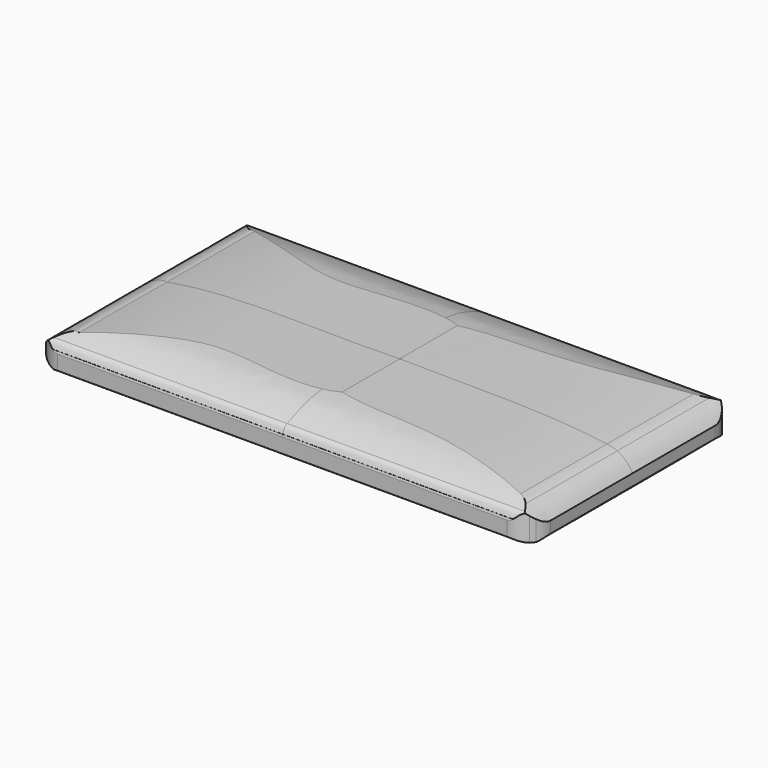
from build123d import *

# Parameters (mm, degrees)
F1_DEPTH = 40
F2_R     = 42.893475334
F3_DEPTH = 77.3
F5_DEPTH = 15


# Not quite as in the source:
# - a feature names something its author has since deleted; it is built from what else it names


with BuildPart() as f1:
    # F0 (on Front) → F1 (new body, symmetric)
    with BuildSketch(Plane.XZ):
        with BuildLine():
            add(Edge.make_bspline(
                [(72.5, -2.7491913643), (72.416496151, -3.810280827), (71.2043847412, -5.7919796052), (69.2787097317, -6.0699322478), (68.1885108352, -6.1267605634)],
                knots=[0, 0, 0, 0, 0.503951183, 1, 1, 1, 1], degree=3))
            add(Edge.make_bspline(
                [(72.5, -2.7491913643), (71.7240370512, -0.9958820883), (70.00554353, 1.4875582419), (67.2821030021, 2.8555840254)],
                knots=[0, 0, 0, 0, 7.657673031, 7.657673031, 7.657673031, 7.657673031], degree=3))
            add(Edge.make_bspline(
                [(67.2821030021, 2.8555840254), (66.6986107826, 3.1973873265), (65.1900321245, 3.5558441274), (64.3139258027, 3.6549806215)],
                knots=[0, 0, 0, 0, 3.0739405988, 3.0739405988, 3.0739405988, 3.0739405988], degree=3))
            add(Edge.make_bspline(
                [(64.3139258027, 3.6549806215), (46.5292930603, 6.1267605634), (25.1828059554, 5.4464280226), (4.5694559813, 5.8230283291)],
                knots=[0, 0, 0, 0, 59.7837946697, 59.7837946697, 59.7837946697, 59.7837946697], degree=3))
            add(Edge.make_bspline(
                [(4.5694559813, 5.8230283291), (-17.8359945615, 5.0541713299), (-41.3991212845, 7.3106954806), (-62.646895647, 3.4530770499)],
                knots=[0, 0, 0, 0, 67.2581191774, 67.2581191774, 67.2581191774, 67.2581191774], degree=3))
            add(Edge.make_bspline(
                [(-62.646895647, 3.4530770499), (-64.7377446294, 3.8790130056), (-69.7105079889, 1.6229992034), (-71.1562633514, -2.3488558363)],
                knots=[0, 0, 0, 0, 10.2991147166, 10.2991147166, 10.2991147166, 10.2991147166], degree=3))
            add(Edge.make_bspline(
                [(-71.1562633514, -2.3488558363), (-70.2665671706, -3.7310614716), (-65.6274408102, -5.3037466102), (-64.372330904, -5.240196883)],
                knots=[0, 0, 0, 0, 7.3743876017, 7.3743876017, 7.3743876017, 7.3743876017], degree=3))
            Line((-64.372330904, -5.240196883), (68.1885108352, -6.1267605634))
        make_face()
    extrude(amount=F1_DEPTH, both=True)

    # F2 (on Right) → F3 (cut, symmetric)
    with BuildSketch(Plane.YZ):
        Circle(F2_R)
        with BuildLine():
            add(Edge.make_bspline(
                [(0, 5.8111241647), (24.4658216834, 6.4411829785), (26.3172594483, 5.8111241584), (34.8840020597, 2.086201217)],
                knots=[0, 0, 0, 0, 35.0823125046, 35.0823125046, 35.0823125046, 35.0823125046], degree=3))
            add(Edge.make_bspline(
                [(34.8840020597, 2.086201217), (35.8897149563, 1.5711296583), (35.8897149563, 1.5711296583), (36.4923961461, 0)],
                knots=[0, 0, 0, 0, 2.6342298789, 2.6342298789, 2.6342298789, 2.6342298789], degree=3))
            add(Edge.make_bspline(
                [(36.4923961461, 0), (36.7086865008, -1.6115957405), (38.0710326135, -4.5721400128), (35.20732373, -5.6221013477)],
                knots=[0, 0, 0, 0, 5.7670993297, 5.7670993297, 5.7670993297, 5.7670993297], degree=3))
            Line((35.20732373, -5.6221013477), (-34.6337743104, -5.6221013477))
            add(Edge.make_bspline(
                [(-34.6337743104, -5.6221013477), (-39.3324792385, -5.1560028987), (-36.3019555807, -0.3326584119), (-36.4923961461, 0)],
                knots=[0, 0, 0, 0, 5.9213595307, 5.9213595307, 5.9213595307, 5.9213595307], degree=3))
            add(Edge.make_bspline(
                [(-34.8840020597, 2.086201217), (-35.8897149563, 1.5711296583), (-35.8897149563, 1.5711296583), (-36.4923961461, 0)],
                knots=[0, 0, 0, 0, 2.6342298789, 2.6342298789, 2.6342298789, 2.6342298789], degree=3))
            add(Edge.make_bspline(
                [(0, 5.8111241647), (-24.4658216834, 6.4411829785), (-26.3172594483, 5.8111241584), (-34.8840020597, 2.086201217)],
                knots=[0, 0, 0, 0, 35.0823125046, 35.0823125046, 35.0823125046, 35.0823125046], degree=3))
        make_face(mode=Mode.SUBTRACT)
    extrude(amount=F3_DEPTH, both=True, mode=Mode.SUBTRACT)

    # F4 (on face) → F5 (cut)
    with BuildSketch(Plane(origin=(0, 0, -5.6221013477), x_dir=(1, 0, 0), z_dir=(0, 0, -1))):
        with BuildLine():
            Line((76.75, -29.65), (76.75, 29.65))
            ThreePointArc((76.75, 29.65), (73.2352813742, 38.1352813742), (64.75, 41.65))
            Line((64.75, 41.65), (-64.75, 41.65))
            ThreePointArc((-64.75, 41.65), (-73.2352813742, 38.1352813742), (-76.75, 29.65))
            Line((-76.75, 29.65), (-76.75, -29.65))
            ThreePointArc((-76.75, -29.65), (-73.2352813742, -38.1352813742), (-64.75, -41.65))
            Line((-64.75, -41.65), (64.75, -41.65))
            ThreePointArc((64.75, -41.65), (73.2352813742, -38.1352813742), (76.75, -29.65))
        make_face()
        with BuildLine():
            Line((-64.75, 36.65), (64.75, 36.65))
            ThreePointArc((64.75, 36.65), (67.4064619165, 36.1263577794), (69.6654850853, 34.6337743104))
            Line((69.6654850853, 34.6337743104), (70.6054432855, 34.6337743104))
            add(Edge.make_bspline(
                [(70.6054432855, 34.6337743104), (70.6054432855, 34.3467944941), (70.6054432855, 34.0598146779), (70.6054432855, 33.7728348617), (70.6054432855, 33.4858550455)],
                knots=[0, 0, 0, 0, 0, 0.0331445032, 0.0331445032, 0.0331445032, 0.0331445032, 0.0331445032], degree=4))
            ThreePointArc((70.6054432855, 33.4858550455), (71.4577605428, 31.6514865727), (71.75, 29.65))
            Line((71.75, 29.65), (71.75, -29.65))
            ThreePointArc((71.75, -29.65), (71.4577605428, -31.6514865727), (70.6054432855, -33.4858550455))
            add(Edge.make_bspline(
                [(70.6054432855, -35.20732373), (70.6054432855, -34.7769565589), (70.6054432855, -34.3465893877), (70.6054432855, -33.9162222166), (70.6054432855, -33.4858550455)],
                knots=[0, 0, 0, 0, 0, 0.0488951864, 0.0488951864, 0.0488951864, 0.0488951864, 0.0488951864], degree=4))
            Line((70.6054432855, -35.20732373), (69.0063074325, -35.20732373))
            ThreePointArc((69.0063074325, -35.20732373), (66.9970796481, -36.2795273629), (64.75, -36.65))
            Line((64.75, -36.65), (-64.75, -36.65))
            ThreePointArc((-64.75, -36.65), (-69.6997474683, -34.5997474683), (-71.75, -29.65))
            Line((-71.75, -29.65), (-71.75, 29.65))
            ThreePointArc((-71.75, 29.65), (-69.6997474683, 34.5997474683), (-64.75, 36.65))
        make_face(mode=Mode.SUBTRACT)
        with BuildLine():
            add(Edge.make_bspline(
                [(70.6054432855, -35.20732373), (70.6054432855, -34.7769565589), (70.6054432855, -34.3465893877), (70.6054432855, -33.9162222166), (70.6054432855, -33.4858550455)],
                knots=[0, 0, 0, 0, 0, 0.0488951864, 0.0488951864, 0.0488951864, 0.0488951864, 0.0488951864], degree=4))
            ThreePointArc((70.6054432855, -33.4858550455), (69.8786196246, -34.4141642232), (69.0063074325, -35.20732373))
            Line((69.0063074325, -35.20732373), (70.6054432855, -35.20732373))
        make_face()
        with BuildLine():
            Line((70.6054432855, 34.6337743104), (69.6654850853, 34.6337743104))
            ThreePointArc((69.6654850853, 34.6337743104), (70.1659629016, 34.0847881402), (70.6054432855, 33.4858550455))
            add(Edge.make_bspline(
                [(70.6054432855, 34.6337743104), (70.6054432855, 34.3467944941), (70.6054432855, 34.0598146779), (70.6054432855, 33.7728348617), (70.6054432855, 33.4858550455)],
                knots=[0, 0, 0, 0, 0, 0.0331445032, 0.0331445032, 0.0331445032, 0.0331445032, 0.0331445032], degree=4))
        make_face()
    extrude(amount=-F5_DEPTH, mode=Mode.SUBTRACT)


solid = f1.part
